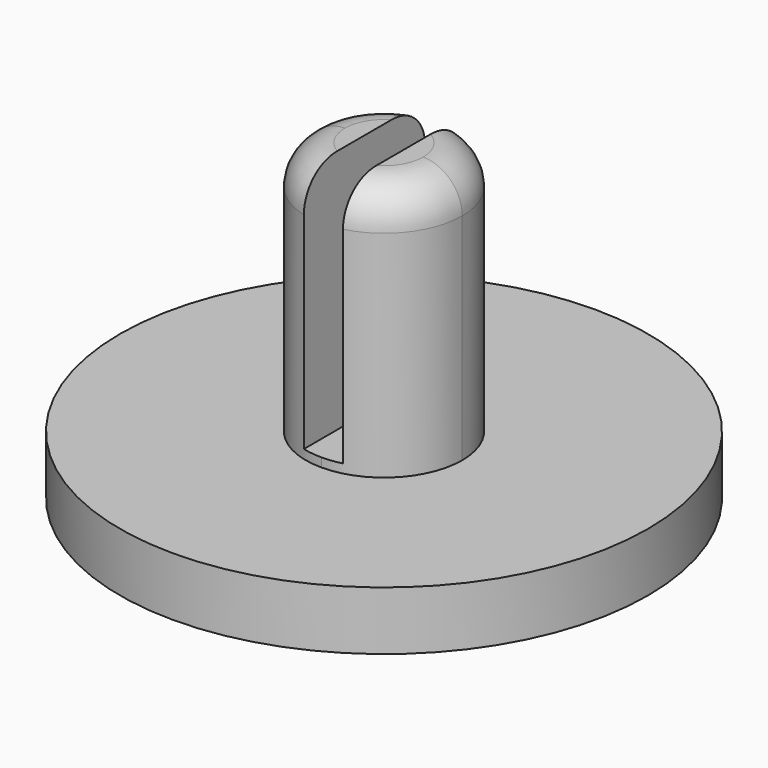
from build123d import *

# Parameters (mm, degrees)
F0_R     = 6.75
F1_DEPTH = 1.5
F2_W     = 4
F2_H     = 4
F3_DEPTH = 6.5
F5_W     = 1
F5_H     = 6.2726680437
F6_DEPTH = 25
F7_R     = 1.99999
F8_R     = 1


# Not quite as in the source:
# - a fillet or chamfer is up to 0.001 mm smaller than in the source, because OpenCascade refuses the exact size


with BuildPart() as f1:
    # F0 (on Top) → F1 (new body)
    with BuildSketch(Plane.XY):
        Circle(F0_R)
    extrude(amount=F1_DEPTH)

    # F2 (on face) → F3 (join)
    with BuildSketch(Plane.XY.offset(1.5)):
        Rectangle(F2_W, F2_H)
    extrude(amount=F3_DEPTH)

    # F5 (on face) → F6 (cut)
    with BuildSketch(Plane.XZ.offset(2)):
        with Locations((0, 4.8636659781)):
            Rectangle(F5_W, F5_H)
    extrude(amount=-F6_DEPTH, mode=Mode.SUBTRACT)

    # F7 (radius 2 in the source; OpenCascade refuses exactly that, so slightly less here)
    f7_edges = [f1.edges().sort_by_distance(p)[0] for p in [
        (2, -2, 4.75),
        (2, 2, 4.75),
        (-2, 2, 4.75),
        (-2, -2, 4.75),
    ]]
    fillet(f7_edges, radius=F7_R)

    # F8
    f8_edges = [f1.edges().sort_by_distance(p)[0] for p in [
        (1.581139, 1.224752, 8),
        (-1.581139, 1.224752, 8),
    ]]
    fillet(f8_edges, radius=F8_R)


solid = f1.part
